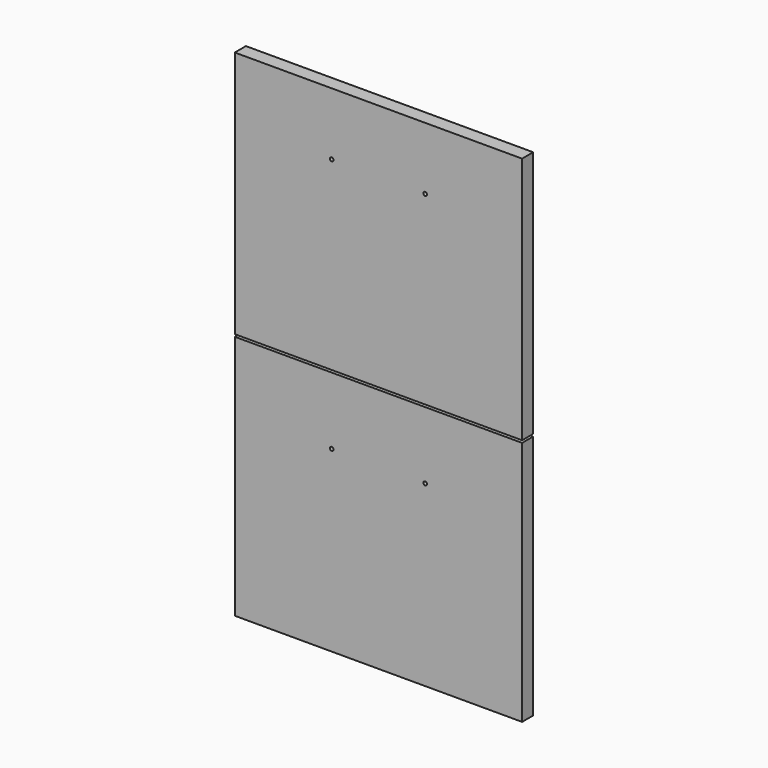
from build123d import *

# Parameters (mm, degrees)
F0_W     = 393.7
F0_H     = 679.45
F1_DEPTH = 19.05
F2_W     = 393.7
F2_H     = 3.175
F3_DEPTH = 25.4
F5_D     = 5.0038
F7_D     = 5.0038


# Not quite as in the source:
# - a feature names something its author has since deleted; it is built from what else it names


with BuildPart() as f1:
    # F0 (on Front) → F1 (new body)
    with BuildSketch(Plane.XZ):
        Rectangle(F0_W, F0_H)
    extrude(amount=F1_DEPTH)

    # F2 (on face) → F3 (cut)
    with BuildSketch(Plane.XZ.offset(19.05)):
        with Locations((0, -1.5875)):
            Rectangle(F2_W, F2_H)
    extrude(amount=-F3_DEPTH, mode=Mode.SUBTRACT)

    # F5 (through all)
    with Locations(Plane.XZ.offset(19.05)):
        with Locations((-64.008, 254), (64.008, 254)):
            Hole(F5_D / 2)

    # F7 (through all)
    with Locations(Plane.XZ.offset(19.05)):
        with Locations((64.008, -95.25), (-64.008, -95.25)):
            Hole(F7_D / 2)


solid = f1.part
